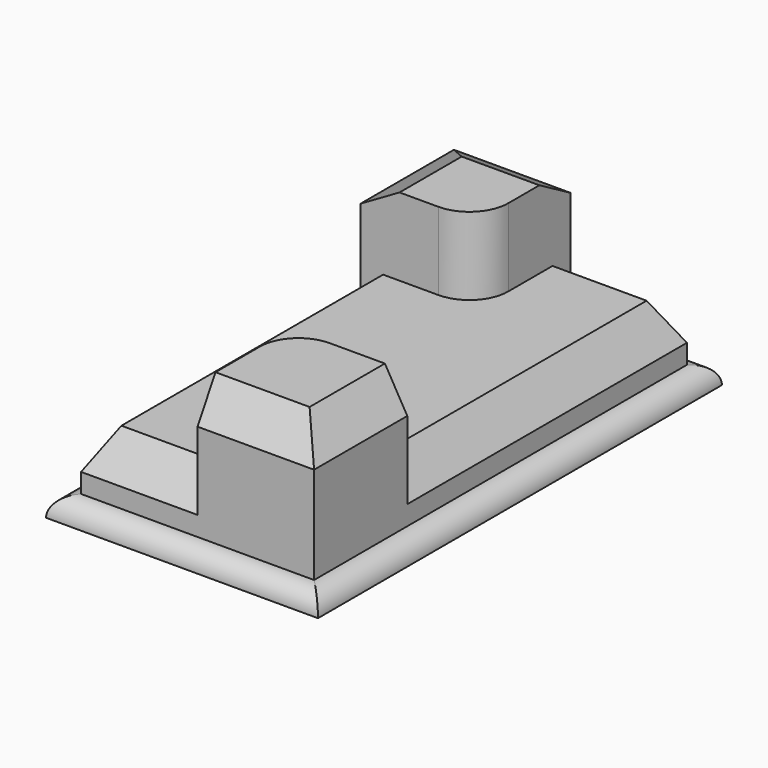
from build123d import *

# Parameters (mm, degrees)
F1_DEPTH    = 25.4
F0_W        = 88.9
F0_H        = 165.1
F2_DEPTH    = 6.35
F3_DEPTH    = 50.8
F4_R        = 6.34999
F5_C1_SIZE2 = 7.3323484187
F5_C1_SIZE  = 12.7
F5_C2_SIZE2 = 12.7
F5_C2_SIZE  = 7.3323484187
F5_C3_SIZE2 = 7.3323484187
F5_C3_SIZE  = 12.7
F5_C4_SIZE2 = 7.3323484187
F5_C4_SIZE  = 12.7
F5_C5_SIZE2 = 7.3323484187
F5_C5_SIZE  = 12.7
F5_C6_SIZE2 = 7.3323484187
F5_C6_SIZE  = 12.7
F5_C7_SIZE2 = 12.7
F5_C7_SIZE  = 7.3323484187
F5_C8_SIZE2 = 7.3323484187
F5_C8_SIZE  = 12.7


# Not quite as in the source:
# - a fillet or chamfer is up to 0.001 mm smaller than in the source, because OpenCascade refuses the exact size


with BuildPart() as f1:
    # F0 (on Top) → F1 (new body)
    with BuildSketch(Plane.XY):
        with BuildLine():
            Line((38.1, -38.1), (38.1, 76.2))
            Line((38.1, 76.2), (0, 76.2))
            Line((0, 76.2), (0, 50.8))
            ThreePointArc((0, 50.8), (-3.7197438789, 41.8197438789), (-12.7, 38.1))
            Line((-12.7, 38.1), (-38.1, 38.1))
            Line((-38.1, 38.1), (-38.1, -76.2))
            Line((-38.1, -76.2), (0, -76.2))
            Line((0, -76.2), (0, -50.8))
            ThreePointArc((0, -50.8), (3.7197438789, -41.8197438789), (12.7, -38.1))
            Line((12.7, -38.1), (38.1, -38.1))
        make_face()
    extrude(amount=F1_DEPTH)

    # F0 (on Top) → F2 (join)
    with BuildSketch(Plane.XY):
        Rectangle(F0_W, F0_H)
        Polygon((0, 76.2), (38.1, 76.2), (38.1, -38.1), (38.1, -76.2), (0, -76.2), (-38.1, -76.2), (-38.1, 38.1), (-38.1, 76.2), align=None, mode=Mode.SUBTRACT)
    extrude(amount=F2_DEPTH)

    # F0 (on Top) → F3 (join)
    with BuildSketch(Plane.XY):
        with BuildLine():
            Line((38.1, -76.2), (38.1, -38.1))
            Line((38.1, -38.1), (12.7, -38.1))
            ThreePointArc((12.7, -38.1), (3.7197438789, -41.8197438789), (0, -50.8))
            Line((0, -50.8), (0, -76.2))
            Line((0, -76.2), (38.1, -76.2))
        make_face()
        with BuildLine():
            Line((0, 50.8), (0, 76.2))
            Line((0, 76.2), (-38.1, 76.2))
            Line((-38.1, 76.2), (-38.1, 38.1))
            Line((-38.1, 38.1), (-12.7, 38.1))
            ThreePointArc((-12.7, 38.1), (-3.7197438789, 41.8197438789), (0, 50.8))
        make_face()
    extrude(amount=F3_DEPTH)

    # F4 (radius 6.35 in the source; OpenCascade refuses exactly that, so slightly less here)
    f4_edges = [f1.edges().sort_by_distance(p)[0] for p in [
        (-44.45, 0, 6.35),
        (0, 82.55, 6.35),
        (44.45, 0, 6.35),
        (0, -82.55, 6.35),
    ]]
    fillet(f4_edges, radius=F4_R)

    # F5: chamfer of 12.7 x 7.3323484187 on 8 edges, made by hand

    # F5_c1
    f5_c1_edges = [f1.edges().sort_by_distance(p)[0] for p in [
        (19.05, 76.2, 25.4),
    ]]
    f5_c1_side = f1.faces().sort_by_distance((19.05, 76.2, 25.2533530316))[0]
    chamfer(f5_c1_edges, length=F5_C1_SIZE, length2=F5_C1_SIZE2, reference=f5_c1_side)

    # F5_c2
    f5_c2_edges = [f1.edges().sort_by_distance(p)[0] for p in [
        (-19.05, 76.2, 50.8),
    ]]
    f5_c2_side = f1.faces().sort_by_distance((-19.05, 76.2, 50.6533530316))[0]
    chamfer(f5_c2_edges, length=F5_C2_SIZE, length2=F5_C2_SIZE2, reference=f5_c2_side)

    # F5_c3
    f5_c3_edges = [f1.edges().sort_by_distance(p)[0] for p in [
        (38.1, -57.15, 50.8),
    ]]
    f5_c3_side = f1.faces().sort_by_distance((38.1, -57.15, 50.6533530316))[0]
    chamfer(f5_c3_edges, length=F5_C3_SIZE, length2=F5_C3_SIZE2, reference=f5_c3_side)

    # F5_c4
    f5_c4_edges = [f1.edges().sort_by_distance(p)[0] for p in [
        (38.1, 15.3838257906, 25.4),
    ]]
    f5_c4_side = f1.faces().sort_by_distance((38.1, 15.3838257906, 25.2533530316))[0]
    chamfer(f5_c4_edges, length=F5_C4_SIZE, length2=F5_C4_SIZE2, reference=f5_c4_side)

    # F5_c5
    f5_c5_edges = [f1.edges().sort_by_distance(p)[0] for p in [
        (-19.05, -76.2, 25.4),
    ]]
    f5_c5_side = f1.faces().sort_by_distance((-19.05, -76.2, 25.2533530316))[0]
    chamfer(f5_c5_edges, length=F5_C5_SIZE, length2=F5_C5_SIZE2, reference=f5_c5_side)

    # F5_c6
    f5_c6_edges = [f1.edges().sort_by_distance(p)[0] for p in [
        (15.3838257906, -76.2, 50.8),
    ]]
    f5_c6_side = f1.faces().sort_by_distance((15.3838257906, -76.2, 50.6533530316))[0]
    chamfer(f5_c6_edges, length=F5_C6_SIZE, length2=F5_C6_SIZE2, reference=f5_c6_side)

    # F5_c7
    f5_c7_edges = [f1.edges().sort_by_distance(p)[0] for p in [
        (-38.1, 50.8, 50.8),
    ]]
    f5_c7_side = f1.faces().sort_by_distance((-38.1, 50.8, 50.6533530316))[0]
    chamfer(f5_c7_edges, length=F5_C7_SIZE, length2=F5_C7_SIZE2, reference=f5_c7_side)

    # F5_c8
    f5_c8_edges = [f1.edges().sort_by_distance(p)[0] for p in [
        (-38.1, -15.3838257906, 25.4),
    ]]
    f5_c8_side = f1.faces().sort_by_distance((-38.1, -15.3838257906, 25.2533530316))[0]
    chamfer(f5_c8_edges, length=F5_C8_SIZE, length2=F5_C8_SIZE2, reference=f5_c8_side)


solid = f1.part
